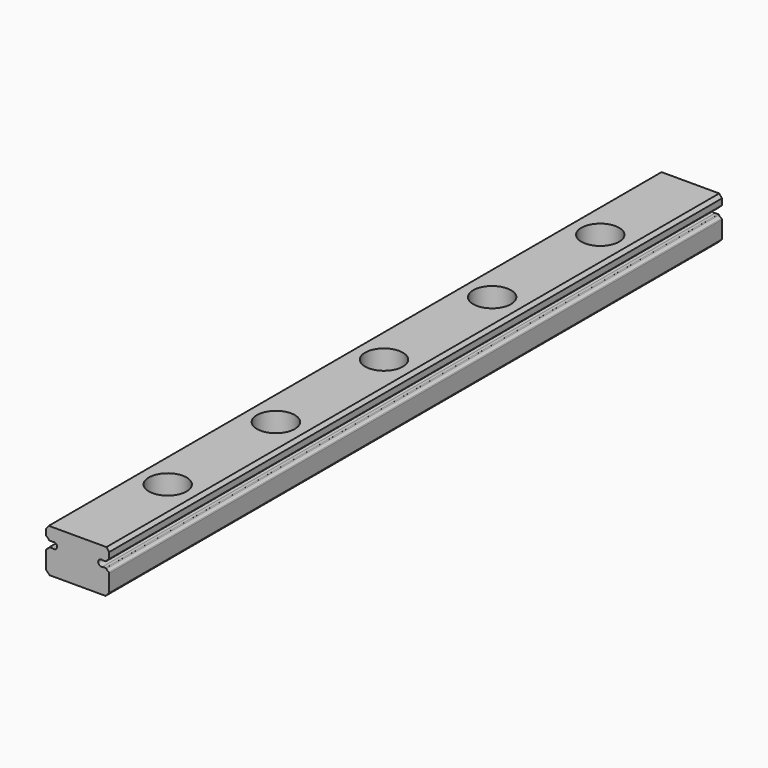
from build123d import *

# Parameters (mm, degrees)
F1_DEPTH       = 42.5
F2_C1_SIZE2    = 0.3
F2_C1_SIZE     = 0.388
F2_C2_SIZE2    = 0.388
F2_C2_SIZE     = 0.3
F3_SIZE        = 0.4
F5_D           = 2.4
F5_CBORE_D     = 4.2
F5_CBORE_DEPTH = 2.3


with BuildPart() as f1:
    # F0 (on Front) → F1 (new body, symmetric)
    with BuildSketch(Plane.XZ):
        with BuildLine():
            Line((-3.5, 0), (3.5, 0))
            Line((3.5, 0), (3.5, 2.3493352987))
            ThreePointArc((3.5, 2.3493352987), (3.4856956825, 2.4008741191), (3.446875, 2.4376683864))
            ThreePointArc((3.446875, 2.4376683864), (3.2976460443, 2.5440105461), (3.1811284368, 2.6854375))
            ThreePointArc((3.1811284368, 2.6854375), (3.1447986618, 2.7199464122), (3.096289642, 2.7325))
            Line((3.096289642, 2.7325), (2.7685954715, 2.7325))
            ThreePointArc((2.7685954715, 2.7325), (2.285, 3.056), (2.7685954715, 3.3795))
            Line((2.7685954715, 3.3795), (3.096289642, 3.3795))
            ThreePointArc((3.096289642, 3.3795), (3.1447986618, 3.3920535878), (3.1811284368, 3.4265625))
            ThreePointArc((3.1811284368, 3.4265625), (3.2976460443, 3.5679894539), (3.446875, 3.6743316136))
            ThreePointArc((3.446875, 3.6743316136), (3.4856956825, 3.7111258809), (3.5, 3.7626647013))
            Line((3.5, 3.7626647013), (3.5, 4.8))
            Line((3.5, 4.8), (-3.5, 4.8))
            Line((-3.5, 4.8), (-3.5, 3.7626647013))
            ThreePointArc((-3.5, 3.7626647013), (-3.4856956825, 3.7111258809), (-3.446875, 3.6743316136))
            ThreePointArc((-3.446875, 3.6743316136), (-3.2976460443, 3.5679894539), (-3.1811284368, 3.4265625))
            ThreePointArc((-3.1811284368, 3.4265625), (-3.1447986618, 3.3920535878), (-3.096289642, 3.3795))
            Line((-3.096289642, 3.3795), (-2.7685954715, 3.3795))
            ThreePointArc((-2.7685954715, 3.3795), (-2.4403958056, 3.3469109959), (-2.285, 3.056))
            ThreePointArc((-2.285, 3.056), (-2.4403958056, 2.7650890041), (-2.7685954715, 2.7325))
            Line((-2.7685954715, 2.7325), (-3.096289642, 2.7325))
            ThreePointArc((-3.096289642, 2.7325), (-3.1447986618, 2.7199464122), (-3.1811284368, 2.6854375))
            ThreePointArc((-3.1811284368, 2.6854375), (-3.2976460443, 2.5440105461), (-3.446875, 2.4376683864))
            ThreePointArc((-3.446875, 2.4376683864), (-3.4856956825, 2.4008741191), (-3.5, 2.3493352987))
            Line((-3.5, 2.3493352987), (-3.5, 0))
        make_face()
    extrude(amount=F1_DEPTH, both=True)

    # F2: chamfer of 0.3 x 0.388 on 2 edges, made by hand

    # F2_c1
    f2_c1_edges = [f1.edges().sort_by_distance(p)[0] for p in [
        (-3.5, 0, 4.8),
    ]]
    f2_c1_side = f1.faces().sort_by_distance((-3.5, 0, 4.794))[0]
    chamfer(f2_c1_edges, length=F2_C1_SIZE, length2=F2_C1_SIZE2, reference=f2_c1_side)

    # F2_c2
    f2_c2_edges = [f1.edges().sort_by_distance(p)[0] for p in [
        (3.5, 0, 4.8),
    ]]
    f2_c2_side = f1.faces().sort_by_distance((3.494, 0, 4.8))[0]
    chamfer(f2_c2_edges, length=F2_C2_SIZE, length2=F2_C2_SIZE2, reference=f2_c2_side)

    # F3
    f3_edges = [f1.edges().sort_by_distance(p)[0] for p in [
        (3.5, 0, 0),
        (-3.5, 0, 0),
    ]]
    chamfer(f3_edges, length=F3_SIZE)

    # F5 (through all)
    with Locations(Plane.XY.offset(4.8)):
        with Locations((0, 30), (0, 15), (0, 0), (0, -15), (0, -30)):
            CounterBoreHole(F5_D / 2, F5_CBORE_D / 2, F5_CBORE_DEPTH)


solid = f1.part
